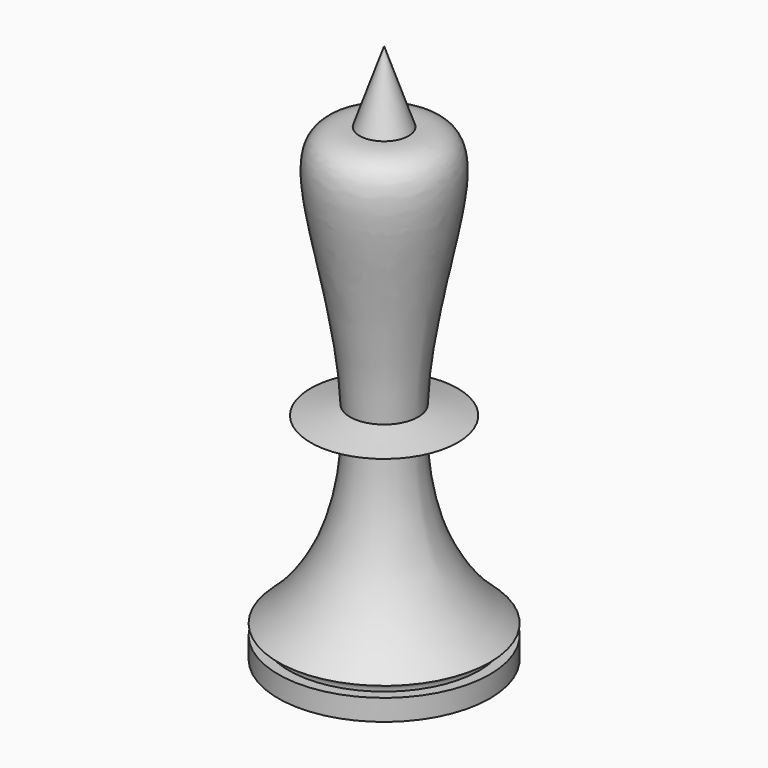
from build123d import *


# Not quite as in the source:
# - a feature names something its author has since deleted; it is built from what else it names


with BuildPart() as f1:
    # F0 (on Front) → F1 (revolve)
    with BuildSketch(Plane.XZ):
        with BuildLine():
            Line((0, 10.7571836561), (0, 0))
            Line((0, 0), (10, 0))
            Line((10, 0), (10, 2))
            Line((10, 2), (9, 2))
            ThreePointArc((9, 2), (9.2928932188, 2.7071067812), (10, 3))
            add(Edge.make_bspline(
                [(10, 3), (4.8616999982, 7.4005079185), (3.2689606671, 13.2153081121), (3.1879616163, 19.0694751767)],
                knots=[0, 0, 0, 0, 0.2884989323, 0.2884989323, 0.2884989323, 0.2884989323], degree=3))
            Line((3.1879616163, 19.0694751767), (0.9205695706, 18.3377522863))
            Line((0.9205695706, 18.3377522863), (0, 10.7571836561))
        make_face()
        with BuildLine():
            Line((0, 51), (0, 44))
            add(Edge.make_bspline(
                [(2.3170218427, 44.2838583015), (1.6508949311, 44.2597847974), (0.8824741052, 44.1653776789), (0, 44)],
                knots=[0.9455867567, 0.9455867567, 0.9455867567, 0.9455867567, 1, 1, 1, 1], degree=3))
            Line((2.3170218427, 44.2838583015), (0, 51))
        make_face()
        with BuildLine():
            Line((1.3255104114, 21.6722985633), (0.9205695706, 18.3377522863))
            Line((0.9205695706, 18.3377522863), (3.1879616163, 19.0694751767))
            add(Edge.make_bspline(
                [(3.1879616163, 19.0694751767), (3.1781161003, 19.7810550677), (3.1906060131, 20.4932165904), (3.2217788711, 21.203490553)],
                knots=[0.2884989323, 0.2884989323, 0.2884989323, 0.2884989323, 0.3235662675, 0.3235662675, 0.3235662675, 0.3235662675], degree=3))
            Line((3.2217788711, 21.203490553), (1.3255104114, 21.6722985633))
        make_face()
        with BuildLine():
            add(Edge.make_bspline(
                [(3.1879616163, 19.0694751767), (3.1781161003, 19.7810550677), (3.1906060131, 20.4932165904), (3.2217788711, 21.203490553)],
                knots=[0.2884989323, 0.2884989323, 0.2884989323, 0.2884989323, 0.3235662675, 0.3235662675, 0.3235662675, 0.3235662675], degree=3))
            Line((3.1879616163, 19.0694751767), (6.9468966685, 20.282542333))
            Line((6.9468966685, 20.282542333), (3.2217788711, 21.203490553))
        make_face()
        with BuildLine():
            Line((1.7987132305, 25.5689583719), (1.3255104114, 21.6722985633))
            Line((1.3255104114, 21.6722985633), (3.2217788711, 21.203490553))
            add(Edge.make_bspline(
                [(3.2217788711, 21.203490553), (3.551315279, 28.7119817542), (7.6075295102, 40.9568023902), (5.393614482, 44.39504487), (2.3170218427, 44.2838583015)],
                knots=[0.3235662675, 0.3235662675, 0.3235662675, 0.3235662675, 0.6942722088, 0.9455867567, 0.9455867567, 0.9455867567, 0.9455867567], degree=3))
            add(Edge.make_bspline(
                [(2.3170218427, 44.2838583015), (1.6508949311, 44.2597847974), (0.8824741052, 44.1653776789), (0, 44)],
                knots=[0.9455867567, 0.9455867567, 0.9455867567, 0.9455867567, 1, 1, 1, 1], degree=3))
            Line((0, 44), (0, 41.3012392819))
            Line((0, 41.3012392819), (3.2213132363, 40.3807349503))
            Line((3.2213132363, 40.3807349503), (3.8907721173, 38.874451071))
            Line((3.8907721173, 38.874451071), (1.7987132305, 25.5689583719))
        make_face()
    revolve(axis=Axis((0, 0, 22), (0, 0, 1)))


solid = f1.part
